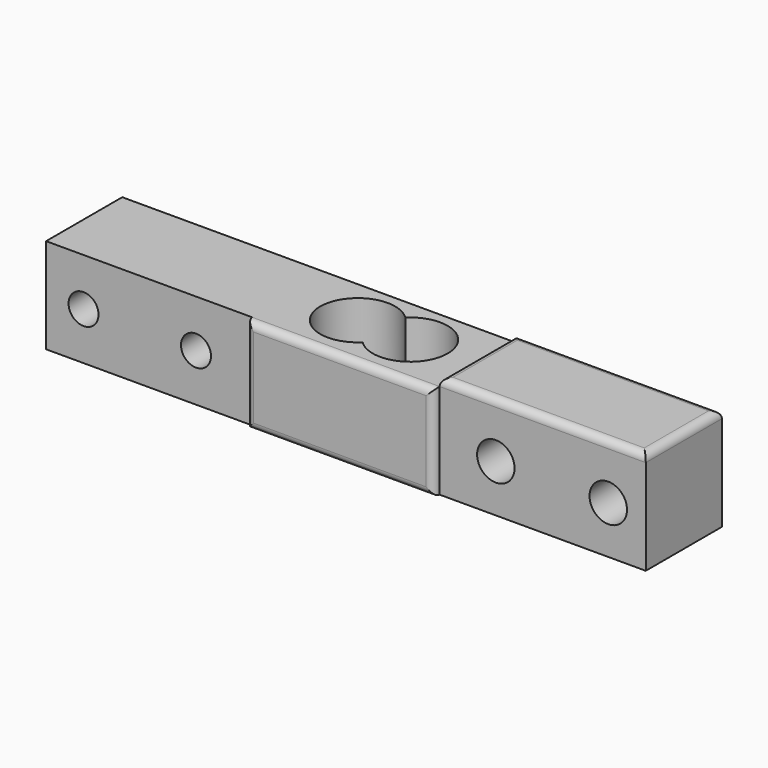
from build123d import *

# Parameters (mm, degrees)
F0_W     = 80
F0_H     = 12.7
F1_DEPTH = 6.35
F2_R     = 2
F2_R_2   = 2.5
F3_DEPTH = 12.701
F5_DEPTH = 12.701
F6_W     = 25
F6_H     = 12.7
F7_DEPTH = 1
F8_W     = 27.5
F8_H     = 12.7
F9_DEPTH = 1
F10_R    = 0.99999


# Not quite as in the source:
# - a fillet or chamfer is up to 0.001 mm smaller than in the source, because OpenCascade refuses the exact size


with BuildPart() as f1:
    # F0 (on Front) → F1 (new body, symmetric)
    with BuildSketch(Plane.XZ):
        Rectangle(F0_W, F0_H)
    extrude(amount=F1_DEPTH, both=True)

    # F2 (on face) → F3 (cut, through all)
    with BuildSketch(Plane.XZ.offset(6.35)):
        with Locations((-35, 0)):
            Circle(F2_R)
        with Locations((-20, 0)):
            Circle(F2_R)
        with Locations((35, 0)):
            Circle(F2_R_2)
        with Locations((20, 0)):
            Circle(F2_R_2)
    extrude(amount=-F3_DEPTH, mode=Mode.SUBTRACT)

    # F4 (on face) → F5 (cut, through all)
    with BuildSketch(Plane.XY.offset(6.35)):
        with BuildLine():
            ThreePointArc((0, -3.5707142143), (5.4364916731, -4.6097722286), (8.5, 0))
            ThreePointArc((8.5, 0), (5.4364916731, 4.6097722286), (0, 3.5707142143))
            ThreePointArc((0, 3.5707142143), (1.1097722286, 1.9364916731), (1.5, 0))
            ThreePointArc((1.5, 0), (1.1097722286, -1.9364916731), (0, -3.5707142143))
        make_face()
        with BuildLine():
            ThreePointArc((1.5, 0), (1.1097722286, 1.9364916731), (0, 3.5707142143))
            ThreePointArc((0, 3.5707142143), (-1.5, 0), (0, -3.5707142143))
            ThreePointArc((0, -3.5707142143), (1.1097722286, -1.9364916731), (1.5, 0))
        make_face()
        with BuildLine():
            ThreePointArc((0, -3.5707142143), (-1.5, 0), (0, 3.5707142143))
            ThreePointArc((0, 3.5707142143), (-8.5, 0), (0, -3.5707142143))
        make_face()
    extrude(amount=-F5_DEPTH, mode=Mode.SUBTRACT)

    # F6 (on face) → F7 (join)
    with BuildSketch(Plane.XZ.offset(6.35)):
        Rectangle(F6_W, F6_H)
    extrude(amount=F7_DEPTH)

    # F8 (on face) → F9 (join)
    with BuildSketch(Plane.XY.offset(6.35)):
        with Locations((26.25, 0)):
            Rectangle(F8_W, F8_H)
    extrude(amount=F9_DEPTH)

    # F10 (radius 1 in the source; OpenCascade refuses exactly that, so slightly less here)
    f10_edges = [f1.edges().sort_by_distance(p)[0] for p in [
        (12.5, 0, 7.35),
        (40, 0, 7.35),
        (0, -7.35, 6.35),
        (0, -7.35, -6.35),
        (12.5, -7.35, 0),
        (-12.5, -7.35, 0),
        (26.25, 6.35, 7.35),
        (26.25, -6.35, 7.35),
    ]]
    fillet(f10_edges, radius=F10_R)


solid = f1.part
